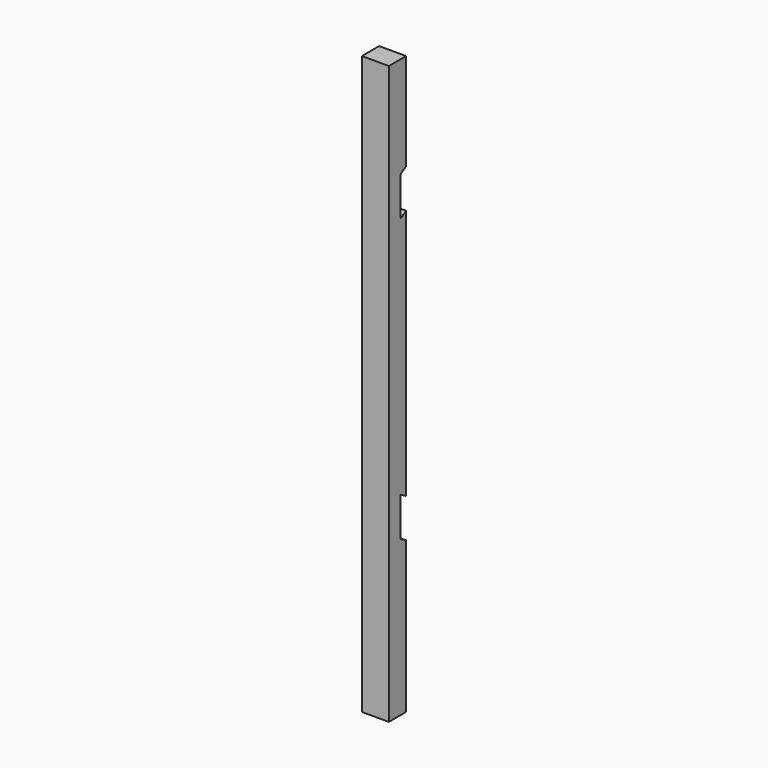
from build123d import *

# Parameters (mm, degrees)
F2_DEPTH = 50


# Not quite as in the source:
# - a feature names something its author has since deleted; it is built from what else it names


with BuildPart() as f2:
    # F1 (on Right) → F2 (new body)
    with BuildSketch(Plane.YZ):
        Polygon((-26.6666666667, 40), (-26.6666666667, 220), (-66.6666666667, 220), (-66.6666666667, -850), (-26.6666666667, -850), (-26.6666666667, -570), (-40, -562.3019964108), (-40, -490), (-26.6666666667, -497.6980035892), (-26.6666666667, -32.3019964108), (-40, -40), (-40, 32.3019964108), align=None)
    extrude(amount=F2_DEPTH)


solid = f2.part
